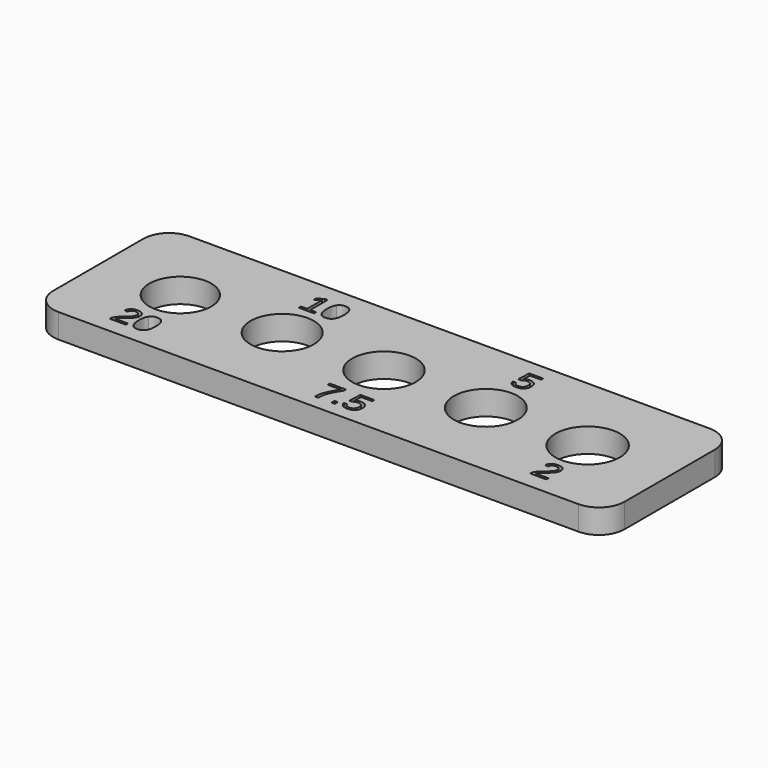
from build123d import *

# Parameters (mm, degrees)
F0_W     = 112.192
F0_H     = 32.192
F0_W_2   = 0.6618923611
F0_H_2   = 0.7421875
F0_R     = 6.096
F0_R_2   = 6.223
F0_R_3   = 6.25475
F0_R_4   = 6.2865
F0_R_5   = 6.3246
F1_DEPTH = 4.7625
F2_R     = 5


# Not quite as in the source:
# - a length typed as a fraction of an inch, garbled in the dataset ("3 / 203.2 mm" for 3/8 in), is restored


with BuildPart() as f1:
    # F0 (on Top) → F1 (new body)
    with BuildSketch(Plane.XY):
        Rectangle(F0_W, F0_H)
        with BuildLine():
            Line((-40.3582831555, -12.9135759734), (-43.5223456555, -12.9135759734))
            Line((-43.5223456555, -12.9135759734), (-43.5223456555, -12.4828034039))
            add(Edge.make_bspline(
                [(-43.5223456555, -12.4828034039), (-43.3498196138, -12.0856679873), (-43.1002536416, -11.7823910775)],
                knots=[0, 0, 0, 1, 1, 1], degree=2))
            add(Edge.make_bspline(
                [(-43.1002536416, -11.7823910775), (-42.8506876694, -11.4791141678), (-42.5761650999, -11.2333459386)],
                knots=[0, 0, 0, 1, 1, 1], degree=2))
            add(Edge.make_bspline(
                [(-42.5761650999, -11.2333459386), (-42.3016425305, -10.9875777095), (-42.0320027735, -10.7770742373)],
                knots=[0, 0, 0, 1, 1, 1], degree=2))
            add(Edge.make_bspline(
                [(-42.0320027735, -10.7770742373), (-41.7623630166, -10.566570765), (-41.5453491277, -10.3566098275)],
                knots=[0, 0, 0, 1, 1, 1], degree=2))
            add(Edge.make_bspline(
                [(-41.5453491277, -10.3566098275), (-41.3283352388, -10.14664889), (-41.1943291624, -9.9160716331)],
                knots=[0, 0, 0, 1, 1, 1], degree=2))
            add(Edge.make_bspline(
                [(-41.1943291624, -9.9160716331), (-41.060323086, -9.6854943761), (-41.060323086, -9.3936106956)],
                knots=[0, 0, 0, 1, 1, 1], degree=2))
            add(Edge.make_bspline(
                [(-41.060323086, -9.3936106956), (-41.060323086, -9.0008155567), (-41.290900343, -8.7838016678)],
                knots=[0, 0, 0, 1, 1, 1], degree=2))
            add(Edge.make_bspline(
                [(-41.290900343, -8.7838016678), (-41.5214775999, -8.5667877789), (-41.9316338499, -8.5667877789)],
                knots=[0, 0, 0, 1, 1, 1], degree=2))
            add(Edge.make_bspline(
                [(-41.9316338499, -8.5667877789), (-42.3222588499, -8.5667877789), (-42.5745374958, -8.7783763206)],
                knots=[0, 0, 0, 1, 1, 1], degree=2))
            add(Edge.make_bspline(
                [(-42.5745374958, -8.7783763206), (-42.8268161416, -8.9899648623), (-42.8713039888, -9.3729943761)],
                knots=[0, 0, 0, 1, 1, 1], degree=2))
            Line((-42.8713039888, -9.3729943761), (-43.4952189194, -9.3154856956))
            add(Edge.make_bspline(
                [(-43.4952189194, -9.3154856956), (-43.4279446138, -8.7425690289), (-43.0091078083, -8.4034848275)],
                knots=[0, 0, 0, 1, 1, 1], degree=2))
            add(Edge.make_bspline(
                [(-43.0091078083, -8.4034848275), (-42.5902710027, -8.0644006261), (-41.9316338499, -8.0644006261)],
                knots=[0, 0, 0, 1, 1, 1], degree=2))
            add(Edge.make_bspline(
                [(-41.9316338499, -8.0644006261), (-41.2100626694, -8.0644006261), (-40.8216078083, -8.4051124317)],
                knots=[0, 0, 0, 1, 1, 1], degree=2))
            add(Edge.make_bspline(
                [(-40.8216078083, -8.4051124317), (-40.4331529472, -8.7458242373), (-40.4331529472, -9.3729943761)],
                knots=[0, 0, 0, 1, 1, 1], degree=2))
            add(Edge.make_bspline(
                [(-40.4331529472, -9.3729943761), (-40.4331529472, -9.6518572234), (-40.5606486069, -9.9263797928)],
                knots=[0, 0, 0, 1, 1, 1], degree=2))
            add(Edge.make_bspline(
                [(-40.5606486069, -9.9263797928), (-40.6881442666, -10.2009023623), (-40.9387953083, -10.4754249317)],
                knots=[0, 0, 0, 1, 1, 1], degree=2))
            add(Edge.make_bspline(
                [(-40.9387953083, -10.4754249317), (-41.1894463499, -10.7499475011), (-41.8979966972, -11.3261193761)],
                knots=[0, 0, 0, 1, 1, 1], degree=2))
            add(Edge.make_bspline(
                [(-41.8979966972, -11.3261193761), (-42.2886216972, -11.6451297928), (-42.5191989541, -11.9012061817)],
                knots=[0, 0, 0, 1, 1, 1], degree=2))
            add(Edge.make_bspline(
                [(-42.5191989541, -11.9012061817), (-42.749776211, -12.1572825706), (-42.8506876694, -12.3949127789)],
                knots=[0, 0, 0, 1, 1, 1], degree=2))
            Line((-42.8506876694, -12.3949127789), (-40.3582831555, -12.3949127789))
            Line((-40.3582831555, -12.3949127789), (-40.3582831555, -12.9135759734))
        make_face(mode=Mode.SUBTRACT)
        with BuildLine():
            add(Edge.make_bspline(
                [(-36.8209567666, -8.6850603484), (-36.4194810722, -9.3057200706), (-36.4194810722, -10.5231679873)],
                knots=[0, 0, 0, 1, 1, 1], degree=2))
            add(Edge.make_bspline(
                [(-36.4194810722, -10.5231679873), (-36.4194810722, -11.7199995845), (-36.841573086, -12.3509674664)],
                knots=[0, 0, 0, 1, 1, 1], degree=2))
            add(Edge.make_bspline(
                [(-36.841573086, -12.3509674664), (-37.2636650999, -12.9819353484), (-38.0872328083, -12.9819353484)],
                knots=[0, 0, 0, 1, 1, 1], degree=2))
            add(Edge.make_bspline(
                [(-38.0872328083, -12.9819353484), (-38.9108005166, -12.9819353484), (-39.3247545097, -12.3542226748)],
                knots=[0, 0, 0, 1, 1, 1], degree=2))
            add(Edge.make_bspline(
                [(-39.3247545097, -12.3542226748), (-39.7387085027, -11.7265100011), (-39.7387085027, -10.5231679873)],
                knots=[0, 0, 0, 1, 1, 1], degree=2))
            add(Edge.make_bspline(
                [(-39.7387085027, -10.5231679873), (-39.7387085027, -9.2916141678), (-39.3366902735, -8.678007397)],
                knots=[0, 0, 0, 1, 1, 1], degree=2))
            add(Edge.make_bspline(
                [(-39.3366902735, -8.678007397), (-38.9346720444, -8.0644006261), (-38.0666164888, -8.0644006261)],
                knots=[0, 0, 0, 1, 1, 1], degree=2))
            add(Edge.make_bspline(
                [(-38.0666164888, -8.0644006261), (-37.222432461, -8.0644006261), (-36.8209567666, -8.6850603484)],
                knots=[0, 0, 0, 1, 1, 1], degree=2))
        make_face(mode=Mode.SUBTRACT)
        with BuildLine():
            Line((-0.5590361603, -8.6450744989), (-0.5590361603, -9.1398661656))
            add(Edge.make_bspline(
                [(-0.5590361603, -9.1398661656), (-1.2914580353, -10.2585727628), (-1.5936498755, -10.8927958531)],
                knots=[0, 0, 0, 1, 1, 1], degree=2))
            add(Edge.make_bspline(
                [(-1.5936498755, -10.8927958531), (-1.8958417158, -11.5270189434), (-2.0466663686, -12.1444234573)],
                knots=[0, 0, 0, 1, 1, 1], degree=2))
            add(Edge.make_bspline(
                [(-2.0466663686, -12.1444234573), (-2.1974910214, -12.7618279712), (-2.1974910214, -13.4226352628)],
                knots=[0, 0, 0, 1, 1, 1], degree=2))
            Line((-2.1974910214, -13.4226352628), (-2.8344267853, -13.4226352628))
            add(Edge.make_bspline(
                [(-2.8344267853, -13.4226352628), (-2.8344267853, -12.5068366517), (-2.4465144589, -11.4950093948)],
                knots=[0, 0, 0, 1, 1, 1], degree=2))
            add(Edge.make_bspline(
                [(-2.4465144589, -11.4950093948), (-2.0586021325, -10.4831821378), (-1.149313938, -9.1637376934)],
                knots=[0, 0, 0, 1, 1, 1], degree=2))
            Line((-1.149313938, -9.1637376934), (-3.7165882436, -9.1637376934))
            Line((-3.7165882436, -9.1637376934), (-3.7165882436, -8.6450744989))
            Line((-3.7165882436, -8.6450744989), (-0.5590361603, -8.6450744989))
        make_face(mode=Mode.SUBTRACT)
        with Locations((0.7538978675, -13.0515415128)):
            Rectangle(F0_W_2, F0_H_2, mode=Mode.SUBTRACT)
        with BuildLine():
            add(Edge.make_bspline(
                [(4.8706513397, -10.7880866517), (5.2894881453, -11.2014981101), (5.2894881453, -11.8666456795)],
                knots=[0, 0, 0, 1, 1, 1], degree=2))
            add(Edge.make_bspline(
                [(5.2894881453, -11.8666456795), (5.2894881453, -12.6218540128), (4.8402693953, -13.0564243253)],
                knots=[0, 0, 0, 1, 1, 1], degree=2))
            add(Edge.make_bspline(
                [(4.8402693953, -13.0564243253), (4.3910506453, -13.4909946378), (3.5935246036, -13.4909946378)],
                knots=[0, 0, 0, 1, 1, 1], degree=2))
            add(Edge.make_bspline(
                [(3.5935246036, -13.4909946378), (2.9262068953, -13.4909946378), (2.5155081106, -13.1991109573)],
                knots=[0, 0, 0, 1, 1, 1], degree=2))
            add(Edge.make_bspline(
                [(2.5155081106, -13.1991109573), (2.1048093259, -12.9072272767), (1.9963023814, -12.3549269295)],
                knots=[0, 0, 0, 1, 1, 1], degree=2))
            Line((1.9963023814, -12.3549269295), (2.6137068953, -12.2833123462))
            add(Edge.make_bspline(
                [(2.6137068953, -12.2833123462), (2.8068492564, -12.9918626934), (3.6076305064, -12.9918626934)],
                knots=[0, 0, 0, 1, 1, 1], degree=2))
            add(Edge.make_bspline(
                [(3.6076305064, -12.9918626934), (4.0991669647, -12.9918626934), (4.3769447425, -12.6950962003)],
                knots=[0, 0, 0, 1, 1, 1], degree=2))
            add(Edge.make_bspline(
                [(4.3769447425, -12.6950962003), (4.6547225203, -12.3983297073), (4.6547225203, -11.8796665128)],
                knots=[0, 0, 0, 1, 1, 1], degree=2))
            add(Edge.make_bspline(
                [(4.6547225203, -11.8796665128), (4.6547225203, -11.4282776239), (4.3753171384, -11.1504998462)],
                knots=[0, 0, 0, 1, 1, 1], degree=2))
            add(Edge.make_bspline(
                [(4.3753171384, -11.1504998462), (4.0959117564, -10.8727220684), (3.6206513397, -10.8727220684)],
                knots=[0, 0, 0, 1, 1, 1], degree=2))
            add(Edge.make_bspline(
                [(3.6206513397, -10.8727220684), (3.3732555064, -10.8727220684), (3.1594968259, -10.9508470684)],
                knots=[0, 0, 0, 1, 1, 1], degree=2))
            add(Edge.make_bspline(
                [(3.1594968259, -10.9508470684), (2.9457381453, -11.0289720684), (2.7319794647, -11.2156040128)],
                knots=[0, 0, 0, 1, 1, 1], degree=2))
            Line((2.7319794647, -11.2156040128), (2.1351912703, -11.2156040128))
            Line((2.1351912703, -11.2156040128), (2.2946964786, -8.6450744989))
            Line((2.2946964786, -8.6450744989), (5.0106252981, -8.6450744989))
            Line((5.0106252981, -8.6450744989), (5.0106252981, -9.1637376934))
            Line((5.0106252981, -9.1637376934), (2.8513371036, -9.1637376934))
            Line((2.8513371036, -9.1637376934), (2.7591062009, -10.6795797073))
            add(Edge.make_bspline(
                [(2.7591062009, -10.6795797073), (3.1562416175, -10.3746751934), (3.7465193953, -10.3746751934)],
                knots=[0, 0, 0, 1, 1, 1], degree=2))
            add(Edge.make_bspline(
                [(3.7465193953, -10.3746751934), (4.4518145342, -10.3746751934), (4.8706513397, -10.7880866517)],
                knots=[0, 0, 0, 1, 1, 1], degree=2))
        make_face(mode=Mode.SUBTRACT)
        with BuildLine():
            Line((42.1094665594, -12.7747418545), (38.9454040594, -12.7747418545))
            Line((38.9454040594, -12.7747418545), (38.9454040594, -12.3439692851))
            add(Edge.make_bspline(
                [(38.9454040594, -12.3439692851), (39.117930101, -11.9468338684), (39.3674960732, -11.6435569587)],
                knots=[0, 0, 0, 1, 1, 1], degree=2))
            add(Edge.make_bspline(
                [(39.3674960732, -11.6435569587), (39.6170620455, -11.340280049), (39.8915846149, -11.0945118198)],
                knots=[0, 0, 0, 1, 1, 1], degree=2))
            add(Edge.make_bspline(
                [(39.8915846149, -11.0945118198), (40.1661071844, -10.8487435906), (40.4357469413, -10.6382401184)],
                knots=[0, 0, 0, 1, 1, 1], degree=2))
            add(Edge.make_bspline(
                [(40.4357469413, -10.6382401184), (40.7053866982, -10.4277366462), (40.9224005871, -10.2177757087)],
                knots=[0, 0, 0, 1, 1, 1], degree=2))
            add(Edge.make_bspline(
                [(40.9224005871, -10.2177757087), (41.139414476, -10.0078147712), (41.2734205524, -9.7772375142)],
                knots=[0, 0, 0, 1, 1, 1], degree=2))
            add(Edge.make_bspline(
                [(41.2734205524, -9.7772375142), (41.4074266288, -9.5466602573), (41.4074266288, -9.2547765767)],
                knots=[0, 0, 0, 1, 1, 1], degree=2))
            add(Edge.make_bspline(
                [(41.4074266288, -9.2547765767), (41.4074266288, -8.8619814379), (41.1768493719, -8.644967549)],
                knots=[0, 0, 0, 1, 1, 1], degree=2))
            add(Edge.make_bspline(
                [(41.1768493719, -8.644967549), (40.9462721149, -8.4279536601), (40.5361158649, -8.4279536601)],
                knots=[0, 0, 0, 1, 1, 1], degree=2))
            add(Edge.make_bspline(
                [(40.5361158649, -8.4279536601), (40.1454908649, -8.4279536601), (39.8932122191, -8.6395422017)],
                knots=[0, 0, 0, 1, 1, 1], degree=2))
            add(Edge.make_bspline(
                [(39.8932122191, -8.6395422017), (39.6409335732, -8.8511307434), (39.596445726, -9.2341602573)],
                knots=[0, 0, 0, 1, 1, 1], degree=2))
            Line((39.596445726, -9.2341602573), (38.9725307955, -9.1766515767))
            add(Edge.make_bspline(
                [(38.9725307955, -9.1766515767), (39.039805101, -8.6037349101), (39.4586419066, -8.2646507087)],
                knots=[0, 0, 0, 1, 1, 1], degree=2))
            add(Edge.make_bspline(
                [(39.4586419066, -8.2646507087), (39.8774787121, -7.9255665073), (40.5361158649, -7.9255665073)],
                knots=[0, 0, 0, 1, 1, 1], degree=2))
            add(Edge.make_bspline(
                [(40.5361158649, -7.9255665073), (41.2576870455, -7.9255665073), (41.6461419066, -8.2662783129)],
                knots=[0, 0, 0, 1, 1, 1], degree=2))
            add(Edge.make_bspline(
                [(41.6461419066, -8.2662783129), (42.0345967677, -8.6069901184), (42.0345967677, -9.2341602573)],
                knots=[0, 0, 0, 1, 1, 1], degree=2))
            add(Edge.make_bspline(
                [(42.0345967677, -9.2341602573), (42.0345967677, -9.5130231045), (41.907101108, -9.787545674)],
                knots=[0, 0, 0, 1, 1, 1], degree=2))
            add(Edge.make_bspline(
                [(41.907101108, -9.787545674), (41.7796054482, -10.0620682434), (41.5289544066, -10.3365908129)],
                knots=[0, 0, 0, 1, 1, 1], degree=2))
            add(Edge.make_bspline(
                [(41.5289544066, -10.3365908129), (41.2783033649, -10.6111133823), (40.5697530177, -11.1872852573)],
                knots=[0, 0, 0, 1, 1, 1], degree=2))
            add(Edge.make_bspline(
                [(40.5697530177, -11.1872852573), (40.1791280177, -11.506295674), (39.9485507607, -11.7623720629)],
                knots=[0, 0, 0, 1, 1, 1], degree=2))
            add(Edge.make_bspline(
                [(39.9485507607, -11.7623720629), (39.7179735038, -12.0184484517), (39.6170620455, -12.2560786601)],
                knots=[0, 0, 0, 1, 1, 1], degree=2))
            Line((39.6170620455, -12.2560786601), (42.1094665594, -12.2560786601))
            Line((42.1094665594, -12.2560786601), (42.1094665594, -12.7747418545))
        make_face(mode=Mode.SUBTRACT)
        with Locations((-40, 0)):
            Circle(F0_R, mode=Mode.SUBTRACT)
        with Locations((-20, 0)):
            Circle(F0_R_2, mode=Mode.SUBTRACT)
        Polygon((-20.1712202364, 8.0504481494), (-23.1649268336, 8.0504481494), (-23.1649268336, 8.5691113439), (-21.9485639864, 8.5691113439), (-21.9485639864, 12.2453266217), (-23.0260379447, 11.4749273161), (-23.0260379447, 12.0521842606), (-21.8975657225, 12.8280089133), (-21.3344146808, 12.8280089133), (-21.3344146808, 8.5691113439), (-20.1712202364, 8.5691113439), align=None, mode=Mode.SUBTRACT)
        with BuildLine():
            add(Edge.make_bspline(
                [(-16.6436594725, 12.2789637744), (-16.242183778, 11.6583040522), (-16.242183778, 10.4408561356)],
                knots=[0, 0, 0, 1, 1, 1], degree=2))
            add(Edge.make_bspline(
                [(-16.242183778, 10.4408561356), (-16.242183778, 9.2440245383), (-16.6642757919, 8.6130566564)],
                knots=[0, 0, 0, 1, 1, 1], degree=2))
            add(Edge.make_bspline(
                [(-16.6642757919, 8.6130566564), (-17.0863678058, 7.9820887744), (-17.9099355141, 7.9820887744)],
                knots=[0, 0, 0, 1, 1, 1], degree=2))
            add(Edge.make_bspline(
                [(-17.9099355141, 7.9820887744), (-18.7335032225, 7.9820887744), (-19.1474572155, 8.6098014481)],
                knots=[0, 0, 0, 1, 1, 1], degree=2))
            add(Edge.make_bspline(
                [(-19.1474572155, 8.6098014481), (-19.5614112086, 9.2375141217), (-19.5614112086, 10.4408561356)],
                knots=[0, 0, 0, 1, 1, 1], degree=2))
            add(Edge.make_bspline(
                [(-19.5614112086, 10.4408561356), (-19.5614112086, 11.672409955), (-19.1593929794, 12.2860167258)],
                knots=[0, 0, 0, 1, 1, 1], degree=2))
            add(Edge.make_bspline(
                [(-19.1593929794, 12.2860167258), (-18.7573747502, 12.8996234967), (-17.8893191947, 12.8996234967)],
                knots=[0, 0, 0, 1, 1, 1], degree=2))
            add(Edge.make_bspline(
                [(-17.8893191947, 12.8996234967), (-17.0451351669, 12.8996234967), (-16.6436594725, 12.2789637744)],
                knots=[0, 0, 0, 1, 1, 1], degree=2))
        make_face(mode=Mode.SUBTRACT)
        Circle(F0_R_3, mode=Mode.SUBTRACT)
        with Locations((20, 0)):
            Circle(F0_R_4, mode=Mode.SUBTRACT)
        with Locations((40, 0)):
            Circle(F0_R_5, mode=Mode.SUBTRACT)
        with BuildLine():
            add(Edge.make_bspline(
                [(20.6452834523, 10.9626682579), (21.0641202579, 10.5492567995), (21.0641202579, 9.8841092301)],
                knots=[0, 0, 0, 1, 1, 1], degree=2))
            add(Edge.make_bspline(
                [(21.0641202579, 9.8841092301), (21.0641202579, 9.1289008968), (20.6149015079, 8.6943305843)],
                knots=[0, 0, 0, 1, 1, 1], degree=2))
            add(Edge.make_bspline(
                [(20.6149015079, 8.6943305843), (20.1656827579, 8.2597602718), (19.3681567162, 8.2597602718)],
                knots=[0, 0, 0, 1, 1, 1], degree=2))
            add(Edge.make_bspline(
                [(19.3681567162, 8.2597602718), (18.7008390079, 8.2597602718), (18.2901402232, 8.5516439523)],
                knots=[0, 0, 0, 1, 1, 1], degree=2))
            add(Edge.make_bspline(
                [(18.2901402232, 8.5516439523), (17.8794414384, 8.8435276329), (17.770934494, 9.3958279801)],
                knots=[0, 0, 0, 1, 1, 1], degree=2))
            Line((17.770934494, 9.3958279801), (18.3883390079, 9.4674425634))
            add(Edge.make_bspline(
                [(18.3883390079, 9.4674425634), (18.581481369, 8.7588922162), (19.382262619, 8.7588922162)],
                knots=[0, 0, 0, 1, 1, 1], degree=2))
            add(Edge.make_bspline(
                [(19.382262619, 8.7588922162), (19.8737990773, 8.7588922162), (20.1515768551, 9.0556587093)],
                knots=[0, 0, 0, 1, 1, 1], degree=2))
            add(Edge.make_bspline(
                [(20.1515768551, 9.0556587093), (20.4293546329, 9.3524252023), (20.4293546329, 9.8710883968)],
                knots=[0, 0, 0, 1, 1, 1], degree=2))
            add(Edge.make_bspline(
                [(20.4293546329, 9.8710883968), (20.4293546329, 10.3224772856), (20.1499492509, 10.6002550634)],
                knots=[0, 0, 0, 1, 1, 1], degree=2))
            add(Edge.make_bspline(
                [(20.1499492509, 10.6002550634), (19.870543869, 10.8780328412), (19.3952834523, 10.8780328412)],
                knots=[0, 0, 0, 1, 1, 1], degree=2))
            add(Edge.make_bspline(
                [(19.3952834523, 10.8780328412), (19.147887619, 10.8780328412), (18.9341289384, 10.7999078412)],
                knots=[0, 0, 0, 1, 1, 1], degree=2))
            add(Edge.make_bspline(
                [(18.9341289384, 10.7999078412), (18.7203702579, 10.7217828412), (18.5066115773, 10.5351508968)],
                knots=[0, 0, 0, 1, 1, 1], degree=2))
            Line((18.5066115773, 10.5351508968), (17.9098233829, 10.5351508968))
            Line((17.9098233829, 10.5351508968), (18.0693285912, 13.1056804106))
            Line((18.0693285912, 13.1056804106), (20.7852574107, 13.1056804106))
            Line((20.7852574107, 13.1056804106), (20.7852574107, 12.5870172162))
            Line((20.7852574107, 12.5870172162), (18.6259692162, 12.5870172162))
            Line((18.6259692162, 12.5870172162), (18.5337383134, 11.0711752023))
            add(Edge.make_bspline(
                [(18.5337383134, 11.0711752023), (18.9308737301, 11.3760797162), (19.5211515079, 11.3760797162)],
                knots=[0, 0, 0, 1, 1, 1], degree=2))
            add(Edge.make_bspline(
                [(19.5211515079, 11.3760797162), (20.2264466468, 11.3760797162), (20.6452834523, 10.9626682579)],
                knots=[0, 0, 0, 1, 1, 1], degree=2))
        make_face(mode=Mode.SUBTRACT)
    extrude(amount=F1_DEPTH)

    # F2
    f2_edges = [f1.edges().sort_by_distance(p)[0] for p in [
        (-56.096, -16.096, 2.38125),
        (-56.096, 16.096, 2.38125),
        (56.096, 16.096, 2.38125),
        (56.096, -16.096, 2.38125),
    ]]
    fillet(f2_edges, radius=F2_R)


solid = f1.part
